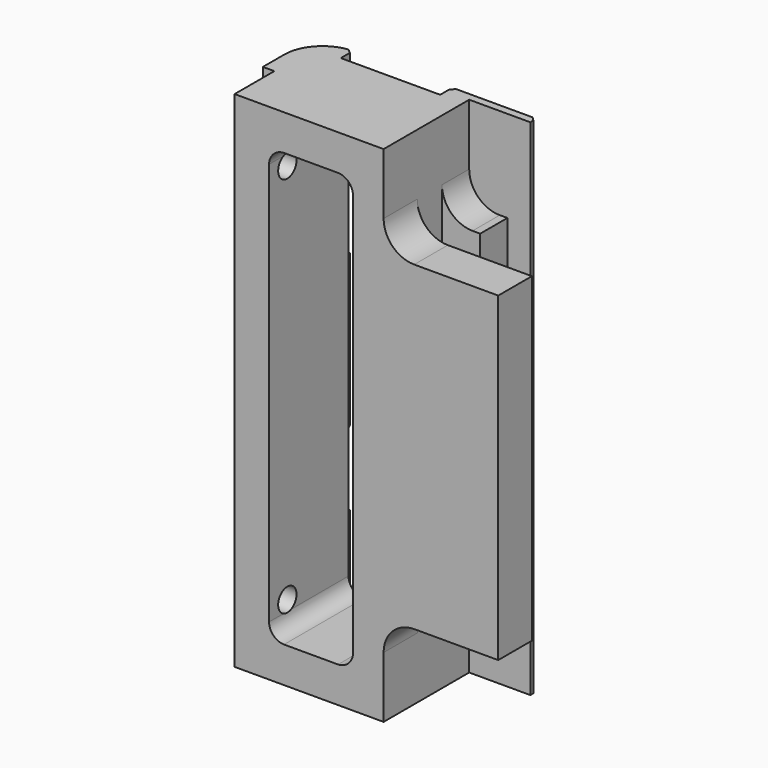
from build123d import *

# Parameters (mm, degrees)
F0_W           = 21
F0_H           = 66
F0_W_2         = 11
F0_H_2         = 56.642
F1_DEPTH       = 15
F2_R           = 5
F4_START       = 9.5
F3_W           = 15
F3_H           = 42
F4_DEPTH       = 5.5
F5_T1_DEPTH    = 15
F6_W           = 1.5
F6_H           = 6.5
F7_DEPTH       = 50
F7_DEPTH_BACK  = 50
F8_R           = 1.5
F9_DEPTH       = 5
F10_W          = 3
F10_H          = 1
F11_DEPTH      = 33
F11_DEPTH_BACK = 33
F12_SIZE       = 0.5
F13_W          = 5
F13_H          = 12
F14_DEPTH      = 14
F15_R          = 4
F16_W          = 13
F16_H          = 70
F17_DEPTH      = 2
F18_W          = 20
F18_H          = 12
F19_DEPTH      = 2
F20_R          = 2
F21_T1_DEPTH   = 68.8536746712
F21_T3_DEPTH   = 11.490341494
F21_T5_DEPTH   = 3
F21_T7_DEPTH   = 8
F21_T9_DEPTH   = 11.490341494
F21_T11_DEPTH  = 13.591
F21_T13_DEPTH  = 8
F21_T16_ANGLE  = 90
F21_T18_ANGLE  = 90
F21_T20_ANGLE  = 90
F21_T22_ANGLE  = 90
F21_T24_ANGLE  = 90
F21_T26_ANGLE  = 90
F21_T28_ANGLE  = 90
F21_T30_ANGLE  = 90
F23_START      = -6.5
F22_R          = 6
F23_DEPTH      = 5.001


# Not quite as in the source:
# - a fillet or chamfer that OpenCascade refuses, or shapes differently, is made with other operations: its cross-section is extruded or revolved along the edge and cut away or added


with BuildPart() as f1:
    # F0 (on Front) → F1 (new body)
    with BuildSketch(Plane.XZ):
        with Locations((-1, 0)):
            Rectangle(F0_W, F0_H)
        Rectangle(F0_W_2, F0_H_2, mode=Mode.SUBTRACT)
    extrude(amount=F1_DEPTH)

    # F2
    f2_edges = [f1.edges().sort_by_distance(p)[0] for p in [
        (-11.5, 0, 0),
    ]]
    fillet(f2_edges, radius=F2_R)

    # F3 (on Front) → F4 (join)
    with BuildSketch(Plane.XZ.offset(F4_START)):
        with Locations((17, 0)):
            Rectangle(F3_W, F3_H)
    extrude(amount=F4_DEPTH)

    # F5: fillet of radius 2 on 4 edges, made by hand

    # F5_s2 → F5_t1 (join)
    with BuildSketch(Plane.XZ):
        with BuildLine():
            ThreePointArc((5.5004, -26.3200343146), (4.9142135624, -27.7352135624), (3.4990343146, -28.3214))
            Line((3.4990343146, -28.3214), (3.4990343146, -28.5215365685))
            ThreePointArc((3.4990343146, -28.5215365685), (4.4995171573, -28.5211365685), (5.5, -28.5211365685))
            Line((5.5, -28.5211365685), (5.7001365685, -28.321))
            ThreePointArc((5.7001365685, -28.321), (5.7001365685, -27.3205171573), (5.7005365685, -26.3200343146))
            Line((5.7005365685, -26.3200343146), (5.5004, -26.3200343146))
        make_face()
        with BuildLine():
            ThreePointArc((-3.4990343146, -28.3214), (-4.9142135624, -27.7352135624), (-5.5004, -26.3200343146))
            Line((-5.5004, -26.3200343146), (-5.7005365685, -26.3200343146))
            ThreePointArc((-5.7005365685, -26.3200343146), (-5.7001365685, -27.3205171573), (-5.7001365685, -28.321))
            Line((-5.7001365685, -28.321), (-5.5, -28.5211365685))
            ThreePointArc((-5.5, -28.5211365685), (-4.4995171573, -28.5211365685), (-3.4990343146, -28.5215365685))
            Line((-3.4990343146, -28.5215365685), (-3.4990343146, -28.3214))
        make_face()
        with BuildLine():
            ThreePointArc((-5.5004, 26.3200343146), (-4.9142135624, 27.7352135624), (-3.4990343146, 28.3214))
            Line((-3.4990343146, 28.3214), (-3.4990343146, 28.5215365685))
            ThreePointArc((-3.4990343146, 28.5215365685), (-4.4995171573, 28.5211365685), (-5.5, 28.5211365685))
            Line((-5.5, 28.5211365685), (-5.7001365685, 28.321))
            ThreePointArc((-5.7001365685, 28.321), (-5.7001365685, 27.3205171573), (-5.7005365685, 26.3200343146))
            Line((-5.7005365685, 26.3200343146), (-5.5004, 26.3200343146))
        make_face()
        with BuildLine():
            ThreePointArc((5.5004, 26.3200343146), (4.9142135624, 27.7352135624), (3.4990343146, 28.3214))
            Line((3.4990343146, 28.3214), (3.4990343146, 28.5215365685))
            ThreePointArc((3.4990343146, 28.5215365685), (4.4995171573, 28.5211365685), (5.5, 28.5211365685))
            Line((5.5, 28.5211365685), (5.7001365685, 28.321))
            ThreePointArc((5.7001365685, 28.321), (5.7001365685, 27.3205171573), (5.7005365685, 26.3200343146))
            Line((5.7005365685, 26.3200343146), (5.5004, 26.3200343146))
        make_face()
    extrude(amount=F5_T1_DEPTH)

    # F6 (on Top) → F7 (cut, two sides)
    with BuildSketch(Plane.XY) as f7_sk:
        with Locations((-10.75, -11.75)):
            Rectangle(F6_W, F6_H)
    extrude(amount=-F7_DEPTH, mode=Mode.SUBTRACT)
    extrude(f7_sk.sketch, amount=F7_DEPTH_BACK, mode=Mode.SUBTRACT)

    # F8 (on face) → F9 (cut)
    with BuildSketch(Plane(origin=(-10, 0, 0), x_dir=(0, -1, 0), z_dir=(-1, 0, 0))):
        with Locations((12, 25)):
            Circle(F8_R)
        with Locations((12, -25)):
            Circle(F8_R)
    extrude(amount=-F9_DEPTH, mode=Mode.SUBTRACT)

    # F10 (on Top) → F11 (join, two sides)
    with BuildSketch(Plane.XY) as f11_sk:
        with Locations((16, -0.5)):
            Rectangle(F10_W, F10_H)
        Polygon((14.5, -5.45), (14.5, -1), (14.5, 0), (9.5, 0), (9.5, -5.45), align=None)
    extrude(amount=F11_DEPTH)
    extrude(f11_sk.sketch, amount=-F11_DEPTH_BACK)

    # F12
    f12_edges = [f1.edges().sort_by_distance(p)[0] for p in [
        (17.5, 0, 0),
    ]]
    chamfer(f12_edges, length=F12_SIZE)

    # F13 (on face) → F14 (cut)
    with BuildSketch(Plane.XZ.offset(15)):
        with Locations((12, -27)):
            Rectangle(F13_W, F13_H)
        with Locations((12, 27)):
            Rectangle(F13_W, F13_H)
    extrude(amount=-F14_DEPTH, mode=Mode.SUBTRACT)

    # F15
    f15_edges = [f1.edges().sort_by_distance(p)[0] for p in [
        (9.5, -3.225, -21),
        (9.5, -12.25, -21),
        (9.5, -3.225, 21),
        (9.5, -12.25, 21),
    ]]
    fillet(f15_edges, radius=F15_R)

    # F16 (on Front) → F17 (cut)
    with BuildSketch(Plane.XZ):
        Rectangle(F16_W, F16_H)
    extrude(amount=F17_DEPTH, mode=Mode.SUBTRACT)

    # F18 (on face) → F19 (cut)
    with BuildSketch(Plane(origin=(0, 0, 0), x_dir=(-1, 0, 0), z_dir=(0, 1, 0))):
        with Locations((-3.5, 14.7955)):
            Rectangle(F18_W, F18_H)
        with Locations((-3.5, -14.7955)):
            Rectangle(F18_W, F18_H)
    extrude(amount=-F19_DEPTH, mode=Mode.SUBTRACT)

    # F20
    f20_edges = [f1.edges().sort_by_distance(p)[0] for p in [
        (13.5, -1, -20.7955),
        (13.5, -1, 20.7955),
        (6.5, -1, 20.7955),
        (6.5, -1, 8.7955),
        (6.5, -1, -8.7955),
        (6.5, -1, -20.7955),
        (13.5, -1, -8.7955),
        (13.5, -1, 8.7955),
    ]]
    fillet(f20_edges, radius=F20_R)

    # F21: chamfer of 0.5 on 18 edges, made by hand

    # F21_s2 → F21_t1 (cut)
    with BuildSketch(Plane.XY.offset(-34.4268373356)):
        with BuildLine():
            Line((-7.0555555556, -0.03096005), (-6.5, -0.527864045))
            Line((-6.5, -0.527864045), (-6.5, 0))
            ThreePointArc((-6.5, 0), (-6.7852695606, -0.0081445055), (-7.0555555556, -0.03096005))
        make_face()
    extrude(amount=F21_T1_DEPTH, mode=Mode.SUBTRACT)

    # F21_s4 → F21_t3 (cut)
    with BuildSketch(Plane.XY.offset(-34.285841494)):
        Polygon((7, 0), (6.5, -0.5), (6.5, 0), align=None)
    extrude(amount=F21_T3_DEPTH, mode=Mode.SUBTRACT)

    # F21_s6 → F21_t5 (cut)
    with BuildSketch(Plane.YZ.offset(8.5)):
        Polygon((0, -21.2955), (-0.5, -20.7955), (0, -20.7955), align=None)
        Polygon((0, -8.2955), (-0.5, -8.7955), (0, -8.7955), align=None)
        Polygon((0, 21.2955), (-0.5, 20.7955), (0, 20.7955), align=None)
        Polygon((0, 8.2955), (-0.5, 8.7955), (0, 8.7955), align=None)
    extrude(amount=F21_T5_DEPTH, mode=Mode.SUBTRACT)

    # F21_s8 → F21_t7 (cut)
    with BuildSketch(Plane.XY.offset(-18.7955)):
        Polygon((14, 0), (13.5, -0.5), (13.5, 0), align=None)
    extrude(amount=F21_T7_DEPTH, mode=Mode.SUBTRACT)

    # F21_s10 → F21_t9 (cut)
    with BuildSketch(Plane.XY.offset(22.7955)):
        Polygon((7, 0), (6.5, -0.5), (6.5, 0), align=None)
    extrude(amount=F21_T9_DEPTH, mode=Mode.SUBTRACT)

    # F21_s12 → F21_t11 (cut)
    with BuildSketch(Plane.XY.offset(-6.7955)):
        Polygon((7, 0), (6.5, -0.5), (6.5, 0), align=None)
    extrude(amount=F21_T11_DEPTH, mode=Mode.SUBTRACT)

    # F21_s14 → F21_t13 (cut)
    with BuildSketch(Plane.XY.offset(10.7955)):
        Polygon((14, 0), (13.5, -0.5), (13.5, 0), align=None)
    extrude(amount=F21_T13_DEPTH, mode=Mode.SUBTRACT)

    # F21_s15 → F21_t16 (revolve, cut)
    with BuildSketch(Plane.YZ.offset(8.5)):
        Polygon((0, -21.2955), (-0.5, -20.7955), (0, -20.7955), align=None)
    revolve(axis=Axis((8.5, 0, -22.7955), (0, -1, 0)), revolution_arc=F21_T16_ANGLE, mode=Mode.SUBTRACT)

    # F21_s17 → F21_t18 (revolve, cut)
    with BuildSketch(Plane.XY.offset(-18.7955)):
        Polygon((14, 0), (13.5, -0.5), (13.5, 0), align=None)
    revolve(axis=Axis((11.5, 0, -18.7955), (0, 1, 0)), revolution_arc=F21_T18_ANGLE, mode=Mode.SUBTRACT)

    # F21_s19 → F21_t20 (revolve, cut)
    with BuildSketch(Plane.YZ.offset(11.5)):
        Polygon((0, -8.2955), (-0.5, -8.7955), (0, -8.7955), align=None)
    revolve(axis=Axis((11.5, 0, -10.7955), (0, 1, 0)), revolution_arc=F21_T20_ANGLE, mode=Mode.SUBTRACT)

    # F21_s21 → F21_t22 (revolve, cut)
    with BuildSketch(Plane.XY.offset(22.7955)):
        Polygon((7, 0), (6.5, -0.5), (6.5, 0), align=None)
    revolve(axis=Axis((8.5, 0, 22.7955), (0, -1, 0)), revolution_arc=F21_T22_ANGLE, mode=Mode.SUBTRACT)

    # F21_s23 → F21_t24 (revolve, cut)
    with BuildSketch(Plane.XY.offset(-6.7955)):
        Polygon((7, 0), (6.5, -0.5), (6.5, 0), align=None)
    revolve(axis=Axis((8.5, 0, -6.7955), (0, -1, 0)), revolution_arc=F21_T24_ANGLE, mode=Mode.SUBTRACT)

    # F21_s25 → F21_t26 (revolve, cut)
    with BuildSketch(Plane.YZ.offset(11.5)):
        Polygon((0, 21.2955), (-0.5, 20.7955), (0, 20.7955), align=None)
    revolve(axis=Axis((11.5, 0, 18.7955), (0, 1, 0)), revolution_arc=F21_T26_ANGLE, mode=Mode.SUBTRACT)

    # F21_s27 → F21_t28 (revolve, cut)
    with BuildSketch(Plane.YZ.offset(8.5)):
        Polygon((0, 8.2955), (-0.5, 8.7955), (0, 8.7955), align=None)
    revolve(axis=Axis((8.5, 0, 6.7955), (0, -1, 0)), revolution_arc=F21_T28_ANGLE, mode=Mode.SUBTRACT)

    # F21_s29 → F21_t30 (revolve, cut)
    with BuildSketch(Plane.XY.offset(10.7955)):
        Polygon((14, 0), (13.5, -0.5), (13.5, 0), align=None)
    revolve(axis=Axis((11.5, 0, 10.7955), (0, 1, 0)), revolution_arc=F21_T30_ANGLE, mode=Mode.SUBTRACT)

    # F22 (on Right) → F23 (cut)
    with BuildSketch(Plane.YZ.offset(F23_START)):
        with Locations((3, -14.7955)):
            Circle(F22_R)
        with Locations((3, 14.7955)):
            Circle(F22_R)
    extrude(amount=-F23_DEPTH, mode=Mode.SUBTRACT)


solid = f1.part
